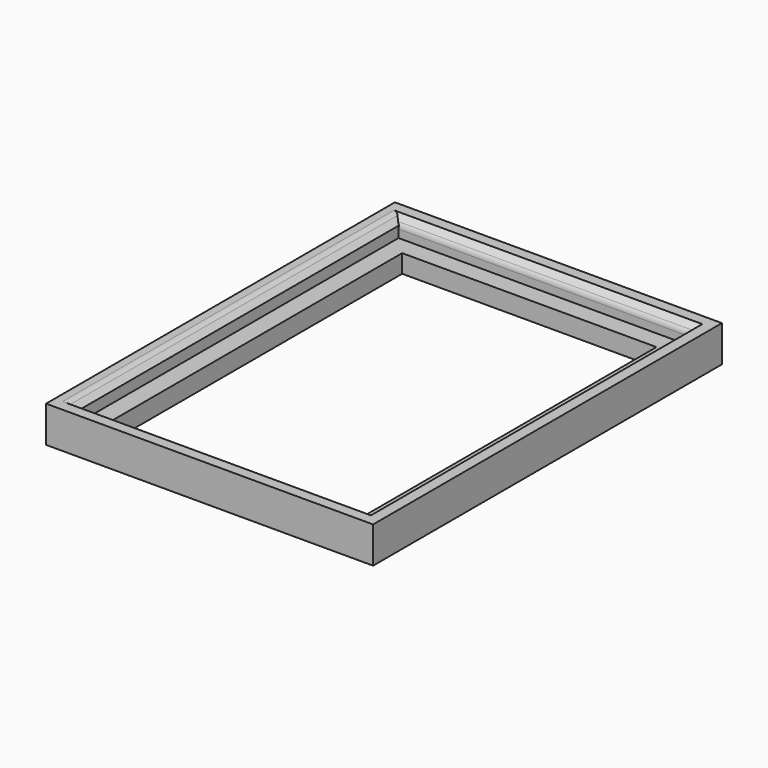
from build123d import *

# Parameters (mm, degrees)
F0_W     = 228.6
F0_H     = 304.8
F0_W_2   = 203.2
F0_H_2   = 279.4
F1_DEPTH = 25.4
F0_W_3   = 177.8
F0_H_3   = 254
F2_DEPTH = 12.7
F3_SIZE  = 5.08
F4_F1_R  = 5.08
F4_F2_R  = 5.08
F4_F3_R  = 5.08
F4_F4_R  = 5.08


with BuildPart() as f1:
    # F0 (on Top) → F1 (new body)
    with BuildSketch(Plane.XY):
        with Locations((114.3, 152.4)):
            Rectangle(F0_W, F0_H)
        with Locations((114.3, 152.4)):
            Rectangle(F0_W_2, F0_H_2, mode=Mode.SUBTRACT)
    extrude(amount=F1_DEPTH)

    # F0 (on Top) → F2 (join)
    with BuildSketch(Plane.XY):
        with Locations((114.3, 152.4)):
            Rectangle(F0_W_2, F0_H_2)
        with Locations((114.3, 152.4)):
            Rectangle(F0_W_3, F0_H_3, mode=Mode.SUBTRACT)
    extrude(amount=F2_DEPTH)

    # F3
    f3_edges = [f1.edges().sort_by_distance(p)[0] for p in [
        (114.3, 292.1, 25.4),
        (215.9, 152.4, 25.4),
        (12.7, 152.4, 25.4),
        (114.3, 12.7, 25.4),
    ]]
    chamfer(f3_edges, length=F3_SIZE)

    # F4: fillet of radius 5.08 on 4 edges, made by hand

    # F4_f1
    f4_f1_edges = [f1.edges().sort_by_distance(p)[0] for p in [
        (7.62, 152.4, 25.4),
    ]]
    fillet(f4_f1_edges, radius=F4_F1_R)

    # F4_f2
    f4_f2_edges = [f1.edges().sort_by_distance(p)[0] for p in [
        (114.3, 292.1, 20.32),
    ]]
    fillet(f4_f2_edges, radius=F4_F2_R)

    # F4_f3
    f4_f3_edges = [f1.edges().sort_by_distance(p)[0] for p in [
        (215.9, 152.6281435083, 20.32),
    ]]
    fillet(f4_f3_edges, radius=F4_F3_R)

    # F4_f4
    f4_f4_edges = [f1.edges().sort_by_distance(p)[0] for p in [
        (114.5281435083, 12.7, 20.32),
    ]]
    fillet(f4_f4_edges, radius=F4_F4_R)


solid = f1.part
